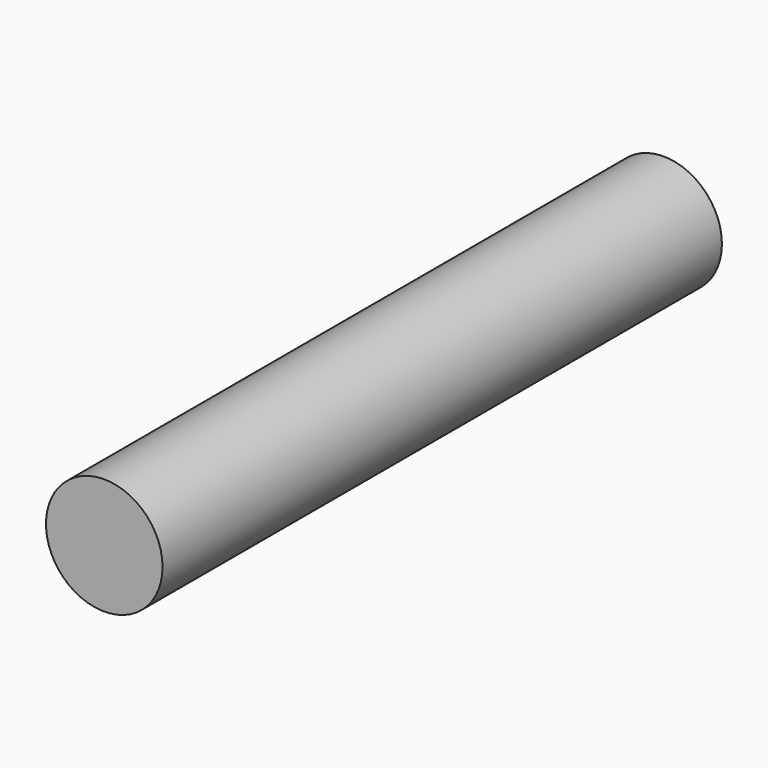
from build123d import *

# Parameters (mm, degrees)
F0_R     = 19.05
F1_DEPTH = 228.6


# Not quite as in the source:
# - the program builds the solid bodies; features that only make, move or delete a surface that nothing else refers to are left out


with BuildPart() as f1:
    # F0 (on Front) → F1 (new body)
    with BuildSketch(Plane.XZ):
        Circle(F0_R)
    extrude(amount=F1_DEPTH)


solid = f1.part
